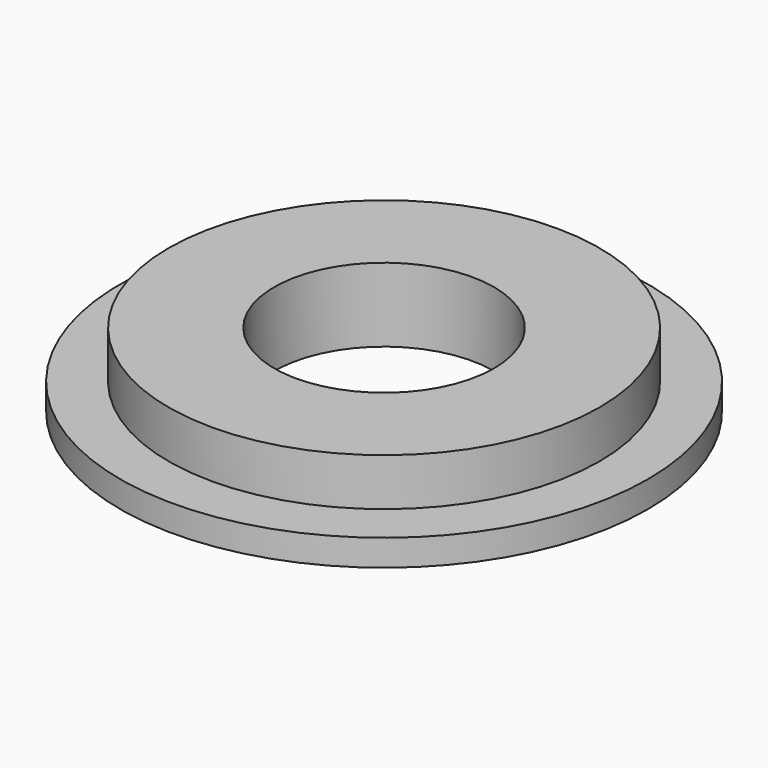
from build123d import *

# Parameters (mm, degrees)
F0_R     = 12.25
F1_DEPTH = 2.7
F2_R     = 15
F2_R_2   = 12.25
F3_DEPTH = 1.5
F4_R     = 6.25
F5_DEPTH = 10


with BuildPart() as f1:
    # F0 (on Top) → F1 (new body)
    with BuildSketch(Plane.XY):
        Circle(F0_R)
    extrude(amount=F1_DEPTH)

    # F2 (on face) → F3 (join)
    with BuildSketch(Plane(origin=(0, 0, 0), x_dir=(1, 0, 0), z_dir=(0, 0, -1))):
        Circle(F2_R)
        Circle(F2_R_2, mode=Mode.SUBTRACT)
        Circle(F2_R_2)
    extrude(amount=F3_DEPTH)

    # F4 (on face) → F5 (cut)
    with BuildSketch(Plane(origin=(0, 0, -1.5), x_dir=(1, 0, 0), z_dir=(0, 0, -1))):
        Circle(F4_R)
    extrude(amount=-F5_DEPTH, mode=Mode.SUBTRACT)


solid = f1.part
